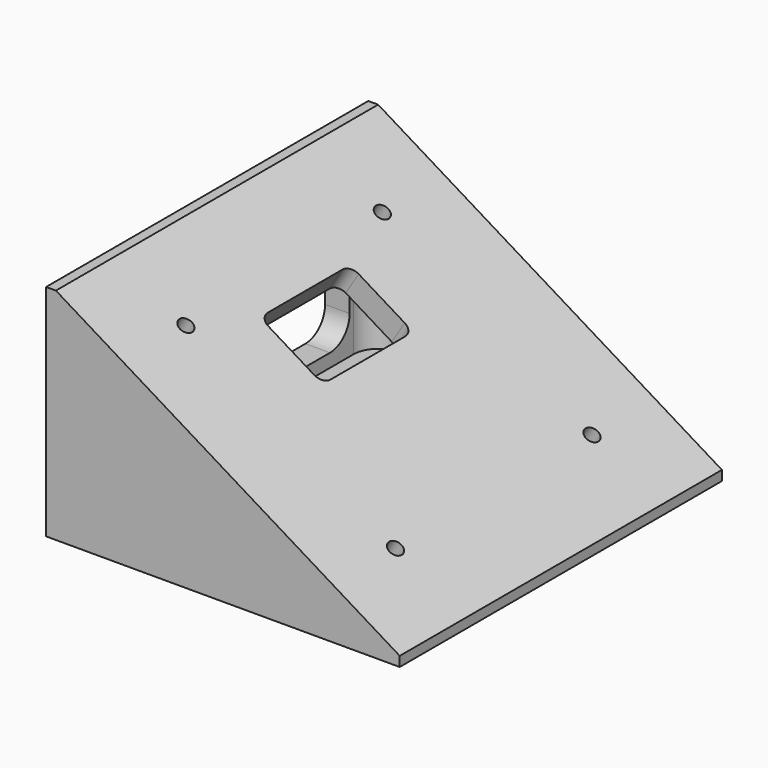
from build123d import *

# Parameters (mm, degrees)
F1_DEPTH  = 104.14
F2_T      = -6.35
F4_D      = 3.81
F4_DEPTH  = 6.604
F4_TIP    = 1.1446394792
F6_DEPTH  = 12.7
F8_DEPTH  = 12.7
F9_R      = 6.35
F10_START = -6.35
F3_R      = 6.35
F10_DEPTH = 19.05
F12_DEPTH = 6.35
F13_D     = 6.5278
F13_DEPTH = 6.604
F13_TIP   = 1.9611489744


with BuildPart() as f1:
    # F0 (on Front) → F1 (new body)
    with BuildSketch(Plane.XZ):
        Polygon((-37.1921509504, 56.5943730235), (-39.7321509504, 56.5943730235), (-39.7321509504, -0.1851844968), (51.7078490496, -0.1851844968), (51.7078490496, 2.3548155032), align=None)
    extrude(amount=-F1_DEPTH)

    # F2 (hollow: no face is removed)
    offset(amount=F2_T, mode=Mode.SUBTRACT)

    # F4
    with Locations(Plane(origin=(15.0736214303, 0, 24.7060449314), x_dir=(0.8536585366, 0, -0.5208330855), z_dir=(0.5208330855, 0, 0.8536585366))):
        with Locations((-40.9056190746, 20.32), (-40.9056190746, 83.82), (22.5943809254, 83.82), (22.5943809254, 20.32)):
            Hole(F4_D / 2, depth=F4_DEPTH)
            with Locations((0, 0, -(F4_DEPTH + F4_TIP / 2))):  # 118° drill point
                Cone(0, F4_D / 2, F4_TIP, mode=Mode.SUBTRACT)

    # F5 (on face) → F6 (cut)
    with BuildSketch(Plane(origin=(15.0736214303, 0, 24.7060449314), x_dir=(0.8536585366, 0, -0.5208330855), z_dir=(0.5208330855, 0, 0.8536585366))):
        with BuildLine():
            ThreePointArc((-34.5556190746, 40.005), (-33.8116702988, 38.2089487758), (-32.0156190746, 37.465))
            Line((-32.0156190746, 37.465), (-18.0456190746, 37.465))
            ThreePointArc((-18.0456190746, 37.465), (-16.2495678504, 38.2089487758), (-15.5056190746, 40.005))
            Line((-15.5056190746, 40.005), (-15.5056190746, 64.135))
            ThreePointArc((-15.5056190746, 64.135), (-16.2495678504, 65.9310512242), (-18.0456190746, 66.675))
            Line((-18.0456190746, 66.675), (-32.0156190746, 66.675))
            ThreePointArc((-32.0156190746, 66.675), (-33.8116702988, 65.9310512242), (-34.5556190746, 64.135))
            Line((-34.5556190746, 64.135), (-34.5556190746, 40.005))
        make_face()
    extrude(amount=-F6_DEPTH, mode=Mode.SUBTRACT)

    # F7 (on face) → F8 (cut)
    with BuildSketch(Plane(origin=(-39.7321509504, 0, 0), x_dir=(0, -1, 0), z_dir=(-1, 0, 0))):
        with BuildLine():
            Line((-20.32, 41.3543730235), (-83.82, 41.3543730235))
            ThreePointArc((-83.82, 41.3543730235), (-88.3101280605, 39.494501084), (-90.17, 35.0043730235))
            Line((-90.17, 35.0043730235), (-90.17, 15.9543730235))
            ThreePointArc((-90.17, 15.9543730235), (-88.3101280605, 11.464244963), (-83.82, 9.6043730235))
            Line((-83.82, 9.6043730235), (-20.32, 9.6043730235))
            ThreePointArc((-20.32, 9.6043730235), (-15.8298719395, 11.464244963), (-13.97, 15.9543730235))
            Line((-13.97, 15.9543730235), (-13.97, 35.0043730235))
            ThreePointArc((-13.97, 35.0043730235), (-15.8298719395, 39.494501084), (-20.32, 41.3543730235))
        make_face()
    extrude(amount=-F8_DEPTH, mode=Mode.SUBTRACT)

    # F9
    f9_edges = [f1.edges().sort_by_distance(p)[0] for p in [
        (-0.055497, 6.35, 26.498032),
        (-0.055497, 97.79, 26.498032),
        (-33.382151, 6.35, 26.498032),
        (-33.382151, 97.79, 26.498032),
    ]]
    fillet(f9_edges, radius=F9_R)

    # F3 (on face) → F10 (cut)
    with BuildSketch(Plane(origin=(15.0736214303, 0, 24.7060449314), x_dir=(0.8536585366, 0, -0.5208330855), z_dir=(0.5208330855, 0, 0.8536585366)).offset(F10_START)):
        with Locations((22.5943809254, 83.82)):
            Circle(F3_R)
        with Locations((22.5943809254, 20.32)):
            Circle(F3_R)
    extrude(amount=-F10_DEPTH, mode=Mode.SUBTRACT)

    # F11 (on face) → F12 (cut)
    with BuildSketch(Plane(origin=(0, 0, -0.1851844968), x_dir=(1, 0, 0), z_dir=(0, 0, -1))):
        with BuildLine():
            ThreePointArc((-5.858374995, -42.1181075931), (-7.7182469345, -37.6279795325), (-12.208374995, -35.7681075931))
            Line((-12.208374995, -35.7681075931), (-18.558374995, -35.7681075931))
            ThreePointArc((-18.558374995, -35.7681075931), (-23.0485030555, -37.6279795325), (-24.908374995, -42.1181075931))
            Line((-24.908374995, -42.1181075931), (-24.908374995, -61.1681075931))
            ThreePointArc((-24.908374995, -61.1681075931), (-23.0485030555, -65.6582356536), (-18.558374995, -67.5181075931))
            Line((-18.558374995, -67.5181075931), (-12.208374995, -67.5181075931))
            ThreePointArc((-12.208374995, -67.5181075931), (-7.7182469345, -65.6582356536), (-5.858374995, -61.1681075931))
            Line((-5.858374995, -61.1681075931), (-5.858374995, -42.1181075931))
        make_face()
    extrude(amount=-F12_DEPTH, mode=Mode.SUBTRACT)

    # F13
    with Locations(Plane(origin=(0, 0, -0.1851844968), x_dir=(1, 0, 0), z_dir=(0, 0, -1))):
        with Locations((5.9878490496, -19.05), (5.9878490496, -85.09)):
            Hole(F13_D / 2, depth=F13_DEPTH)
            with Locations((0, 0, -(F13_DEPTH + F13_TIP / 2))):  # 118° drill point
                Cone(0, F13_D / 2, F13_TIP, mode=Mode.SUBTRACT)


solid = f1.part
